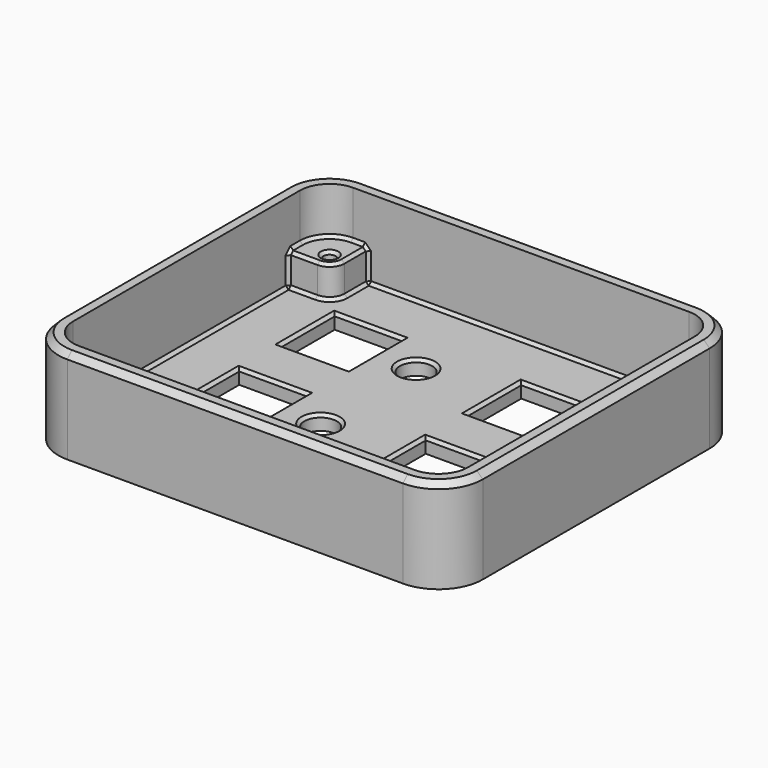
from build123d import *

# Parameters (mm, degrees)
F0_R     = 1
F1_DEPTH = 16
F2_T     = -2.5
F3_DEPTH = 8
F4_W     = 41.64
F4_H     = 10.8
F4_W_2   = 11.5
F4_H_2   = 11.5
F4_R     = 2.75
F5_DEPTH = 2.501
F6_SIZE  = 1
F7_SIZE  = 0.5


with BuildPart() as f1:
    # F0 (on Top) → F1 (new body)
    with BuildSketch(Plane.XY):
        with BuildLine():
            ThreePointArc((-36.115, -24.13), (-33.9065851301, -29.4615851301), (-28.575, -31.67))
            Line((-28.575, -31.67), (-26.035, -31.67))
            Line((-26.035, -31.67), (-26.035, -24.13))
            ThreePointArc((-26.035, -24.13), (-26.7789487758, -22.3339487758), (-28.575, -21.59))
            Line((-28.575, -21.59), (-36.115, -21.59))
            Line((-36.115, -21.59), (-36.115, -24.13))
        make_face()
        with Locations((-28.575, -24.13)):
            Circle(F0_R, mode=Mode.SUBTRACT)
        with BuildLine():
            Line((-26.035, -24.13), (-26.035, -31.67))
            Line((-26.035, -31.67), (26.035, -31.67))
            Line((26.035, -31.67), (26.035, -24.13))
            ThreePointArc((26.035, -24.13), (26.7789487758, -22.3339487758), (28.575, -21.59))
            Line((28.575, -21.59), (36.115, -21.59))
            Line((36.115, -21.59), (36.115, 21.59))
            Line((36.115, 21.59), (28.575, 21.59))
            ThreePointArc((28.575, 21.59), (26.7789487758, 22.3339487758), (26.035, 24.13))
            Line((26.035, 24.13), (26.035, 31.67))
            Line((26.035, 31.67), (-26.035, 31.67))
            Line((-26.035, 31.67), (-26.035, 24.13))
            ThreePointArc((-26.035, 24.13), (-26.7789487758, 22.3339487758), (-28.575, 21.59))
            Line((-28.575, 21.59), (-36.115, 21.59))
            Line((-36.115, 21.59), (-36.115, -21.59))
            Line((-36.115, -21.59), (-28.575, -21.59))
            ThreePointArc((-28.575, -21.59), (-26.7789487758, -22.3339487758), (-26.035, -24.13))
        make_face()
        with BuildLine():
            Line((-36.115, 24.13), (-36.115, 21.59))
            Line((-36.115, 21.59), (-28.575, 21.59))
            ThreePointArc((-28.575, 21.59), (-26.7789487758, 22.3339487758), (-26.035, 24.13))
            Line((-26.035, 24.13), (-26.035, 31.67))
            Line((-26.035, 31.67), (-28.575, 31.67))
            ThreePointArc((-28.575, 31.67), (-33.9065851301, 29.4615851301), (-36.115, 24.13))
        make_face()
        with Locations((-28.575, 24.13)):
            Circle(F0_R, mode=Mode.SUBTRACT)
        with BuildLine():
            Line((26.035, -24.13), (26.035, -31.67))
            Line((26.035, -31.67), (28.575, -31.67))
            ThreePointArc((28.575, -31.67), (33.9065851301, -29.4615851301), (36.115, -24.13))
            Line((36.115, -24.13), (36.115, -21.59))
            Line((36.115, -21.59), (28.575, -21.59))
            ThreePointArc((28.575, -21.59), (26.7789487758, -22.3339487758), (26.035, -24.13))
        make_face()
        with Locations((28.575, -24.13)):
            Circle(F0_R, mode=Mode.SUBTRACT)
        with BuildLine():
            Line((28.575, 21.59), (36.115, 21.59))
            Line((36.115, 21.59), (36.115, 24.13))
            ThreePointArc((36.115, 24.13), (33.9065851301, 29.4615851301), (28.575, 31.67))
            Line((28.575, 31.67), (26.035, 31.67))
            Line((26.035, 31.67), (26.035, 24.13))
            ThreePointArc((26.035, 24.13), (26.7789487758, 22.3339487758), (28.575, 21.59))
        make_face()
        with Locations((28.575, 24.13)):
            Circle(F0_R, mode=Mode.SUBTRACT)
        with Locations((28.575, -24.13)):
            Circle(F0_R)
        with Locations((28.575, 24.13)):
            Circle(F0_R)
        with Locations((-28.575, -24.13)):
            Circle(F0_R)
        with Locations((-28.575, 24.13)):
            Circle(F0_R)
    extrude(amount=F1_DEPTH)

    # F2
    f2_openings = [f1.faces().sort_by_distance(p)[0] for p in [
        (0, 0, 16),
    ]]
    offset(amount=F2_T, openings=f2_openings)

    # F0 (on Top) → F3 (join)
    with BuildSketch(Plane.XY):
        with BuildLine():
            Line((26.035, -24.13), (26.035, -31.67))
            Line((26.035, -31.67), (28.575, -31.67))
            ThreePointArc((28.575, -31.67), (33.9065851301, -29.4615851301), (36.115, -24.13))
            Line((36.115, -24.13), (36.115, -21.59))
            Line((36.115, -21.59), (28.575, -21.59))
            ThreePointArc((28.575, -21.59), (26.7789487758, -22.3339487758), (26.035, -24.13))
        make_face()
        with Locations((28.575, -24.13)):
            Circle(F0_R, mode=Mode.SUBTRACT)
        with BuildLine():
            Line((28.575, 21.59), (36.115, 21.59))
            Line((36.115, 21.59), (36.115, 24.13))
            ThreePointArc((36.115, 24.13), (33.9065851301, 29.4615851301), (28.575, 31.67))
            Line((28.575, 31.67), (26.035, 31.67))
            Line((26.035, 31.67), (26.035, 24.13))
            ThreePointArc((26.035, 24.13), (26.7789487758, 22.3339487758), (28.575, 21.59))
        make_face()
        with Locations((28.575, 24.13)):
            Circle(F0_R, mode=Mode.SUBTRACT)
        with BuildLine():
            Line((-36.115, 24.13), (-36.115, 21.59))
            Line((-36.115, 21.59), (-28.575, 21.59))
            ThreePointArc((-28.575, 21.59), (-26.7789487758, 22.3339487758), (-26.035, 24.13))
            Line((-26.035, 24.13), (-26.035, 31.67))
            Line((-26.035, 31.67), (-28.575, 31.67))
            ThreePointArc((-28.575, 31.67), (-33.9065851301, 29.4615851301), (-36.115, 24.13))
        make_face()
        with Locations((-28.575, 24.13)):
            Circle(F0_R, mode=Mode.SUBTRACT)
        with BuildLine():
            ThreePointArc((-36.115, -24.13), (-33.9065851301, -29.4615851301), (-28.575, -31.67))
            Line((-28.575, -31.67), (-26.035, -31.67))
            Line((-26.035, -31.67), (-26.035, -24.13))
            ThreePointArc((-26.035, -24.13), (-26.7789487758, -22.3339487758), (-28.575, -21.59))
            Line((-28.575, -21.59), (-36.115, -21.59))
            Line((-36.115, -21.59), (-36.115, -24.13))
        make_face()
        with Locations((-28.575, -24.13)):
            Circle(F0_R, mode=Mode.SUBTRACT)
    extrude(amount=F3_DEPTH)

    # F4 (on face) → F5 (cut, through all)
    with BuildSketch(Plane.XY.offset(2.5)):
        with Locations((0.365, -19.16)):
            Rectangle(F4_W, F4_H)
        with Locations((-18.415, 13.97)):
            Rectangle(F4_W_2, F4_H_2)
        with Locations((-5.715, 13.97)):
            Circle(F4_R)
        with Locations((-18.415, -6.35)):
            Rectangle(F4_W_2, F4_H_2)
        with Locations((-5.715, -6.35)):
            Circle(F4_R)
        with Locations((13.335, 13.97)):
            Rectangle(F4_W_2, F4_H_2)
        with Locations((26.035, 13.97)):
            Circle(F4_R)
        with Locations((13.335, -6.35)):
            Rectangle(F4_W_2, F4_H_2)
        with Locations((26.035, -6.35)):
            Circle(F4_R)
    extrude(amount=-F5_DEPTH, mode=Mode.SUBTRACT)

    # F6
    f6_edges = [f1.edges().sort_by_distance(p)[0] for p in [
        (-36.115, 0, 16),
        (-33.906585, -29.461585, 16),
        (0, -31.67, 16),
        (33.906585, -29.461585, 16),
        (36.115, 0, 16),
        (33.906585, 29.461585, 16),
        (0, 31.67, 16),
        (-33.906585, 29.461585, 16),
    ]]
    chamfer(f6_edges, length=F6_SIZE)

    # F7
    f7_edges = [f1.edges().sort_by_distance(p)[0] for p in [
        (-33.615, 22.86, 8),
        (-32.138818, 27.693818, 8),
        (-27.305, 29.17, 8),
        (-26.035, 26.65, 8),
        (-26.778949, 22.333949, 8),
        (-31.095, 21.59, 8),
        (-29.575, 24.13, 8),
        (26.778949, 22.333949, 8),
        (26.035, 26.65, 8),
        (27.305, 29.17, 8),
        (32.138818, 27.693818, 8),
        (33.615, 22.86, 8),
        (31.095, 21.59, 8),
        (27.575, 24.13, 8),
        (26.778949, -22.333949, 8),
        (31.095, -21.59, 8),
        (33.615, -22.86, 8),
        (32.138818, -27.693818, 8),
        (27.305, -29.17, 8),
        (26.035, -26.65, 8),
        (27.575, -24.13, 8),
        (-31.095, -21.59, 8),
        (-26.778949, -22.333949, 8),
        (-26.035, -26.65, 8),
        (-27.305, -29.17, 8),
        (-32.138818, -27.693818, 8),
        (-33.615, -22.86, 8),
        (-29.575, -24.13, 8),
        (-26.035, -26.65, 2.5),
        (-26.778949, -22.333949, 2.5),
        (0, -29.17, 2.5),
        (-31.095, -21.59, 2.5),
        (26.035, -26.65, 2.5),
        (-33.615, 0, 2.5),
        (26.778949, -22.333949, 2.5),
        (-31.095, 21.59, 2.5),
        (31.095, -21.59, 2.5),
        (-26.778949, 22.333949, 2.5),
        (33.615, 0, 2.5),
        (-26.035, 26.65, 2.5),
        (31.095, 21.59, 2.5),
        (0, 29.17, 2.5),
        (26.778949, 22.333949, 2.5),
        (26.035, 26.65, 2.5),
        (0.365, -13.76, 2.5),
        (-20.455, -19.16, 2.5),
        (0.365, -24.56, 2.5),
        (21.185, -19.16, 2.5),
        (-12.665, -6.35, 2.5),
        (-18.415, -0.6, 2.5),
        (-24.165, -6.35, 2.5),
        (-18.415, -12.1, 2.5),
        (-8.465, -6.35, 2.5),
        (13.335, -12.1, 2.5),
        (19.085, -6.35, 2.5),
        (13.335, -0.6, 2.5),
        (7.585, -6.35, 2.5),
        (23.285, -6.35, 2.5),
        (-12.665, 13.97, 2.5),
        (-18.415, 19.72, 2.5),
        (-24.165, 13.97, 2.5),
        (-18.415, 8.22, 2.5),
        (-8.465, 13.97, 2.5),
        (13.335, 8.22, 2.5),
        (19.085, 13.97, 2.5),
        (13.335, 19.72, 2.5),
        (7.585, 13.97, 2.5),
        (23.285, 13.97, 2.5),
        (-33.615, 21.59, 5.25),
        (-33.615, -21.59, 5.25),
        (26.035, 29.17, 5.25),
        (-26.035, 29.17, 5.25),
        (33.615, -21.59, 5.25),
        (33.615, 21.59, 5.25),
        (-26.035, -29.17, 5.25),
        (26.035, -29.17, 5.25),
    ]]
    chamfer(f7_edges, length=F7_SIZE)


solid = f1.part
